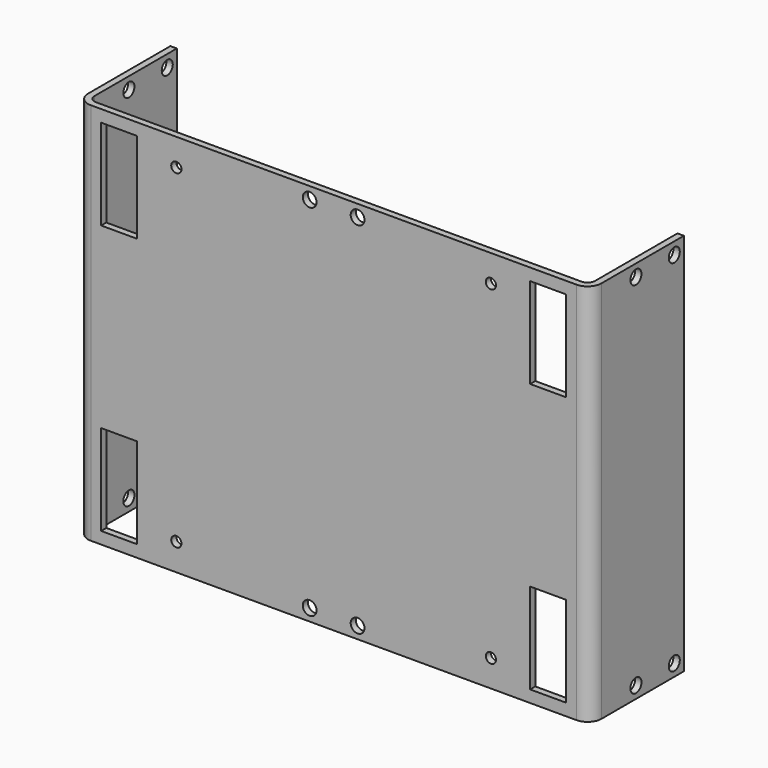
from build123d import *

# Parameters (mm, degrees)
F1_DEPTH = 101.6
F2_R     = 1.98374
F3_R     = 3.69316
F4_W     = 9.5329248
F4_H     = 24
F4_R     = 1.35255
F4_R_2   = 1.8288
F5_DEPTH = 257
F6_R     = 1.8288
F7_DEPTH = 136.06526


# Not quite as in the source:
# - an extrude ends at something that could not be found from the text; its depth is read off the source's solid


with BuildPart() as f1:
    # F0 (on Top) → F1 (new body)
    with BuildSketch(Plane.XY):
        Polygon((0, 29.2656006), (0, 0), (-132.64642, 0), (-132.64642, 29.2656006), (-134.35584, 29.2656006), (-134.35584, -1.70942), (1.70942, -1.70942), (1.70942, 29.2656006), align=None)
    extrude(amount=F1_DEPTH)

    # F2
    f2_edges = [f1.edges().sort_by_distance(p)[0] for p in [
        (0, 0, 50.8),
        (-132.64642, 0, 50.8),
    ]]
    fillet(f2_edges, radius=F2_R)

    # F3
    f3_edges = [f1.edges().sort_by_distance(p)[0] for p in [
        (-134.35584, -1.70942, 50.8),
        (1.70942, -1.70942, 50.8),
    ]]
    fillet(f3_edges, radius=F3_R)

    # F4 (on face) → F5 (cut, through all)
    with BuildSketch(Plane.XZ.offset(1.70942)):
        with Locations((-9.48374, 15.175)):
            Rectangle(F4_W, F4_H)
        with Locations((-123.16268, 15.175)):
            Rectangle(F4_W, F4_H)
        with Locations((-123.16268, 86.425)):
            Rectangle(F4_W, F4_H)
        with Locations((-9.48374, 86.425)):
            Rectangle(F4_W, F4_H)
        with Locations((-24.6456604, 7.14375)):
            Circle(F4_R)
        with Locations((-108.0007596, 7.14375)):
            Circle(F4_R)
        with Locations((-108.0007596, 94.45625)):
            Circle(F4_R)
        with Locations((-24.6456604, 94.45625)):
            Circle(F4_R)
        with Locations((-59.97321, 3.175)):
            Circle(F4_R_2)
        with Locations((-72.67321, 3.175)):
            Circle(F4_R_2)
        with Locations((-59.97321, 98.425)):
            Circle(F4_R_2)
        with Locations((-72.67321, 98.425)):
            Circle(F4_R_2)
    extrude(amount=-F5_DEPTH, mode=Mode.SUBTRACT)

    # F6 (on face) → F7 (cut, through all)
    with BuildSketch(Plane(origin=(-134.35584, 0, 0), x_dir=(0, -1, 0), z_dir=(-1, 0, 0))):
        with Locations((-26.0906006, 3.175)):
            Circle(F6_R)
        with Locations((-13.3906006, 3.175)):
            Circle(F6_R)
        with Locations((-13.3906006, 98.425)):
            Circle(F6_R)
        with Locations((-26.0906006, 98.425)):
            Circle(F6_R)
    extrude(amount=-F7_DEPTH, mode=Mode.SUBTRACT)


solid = f1.part
